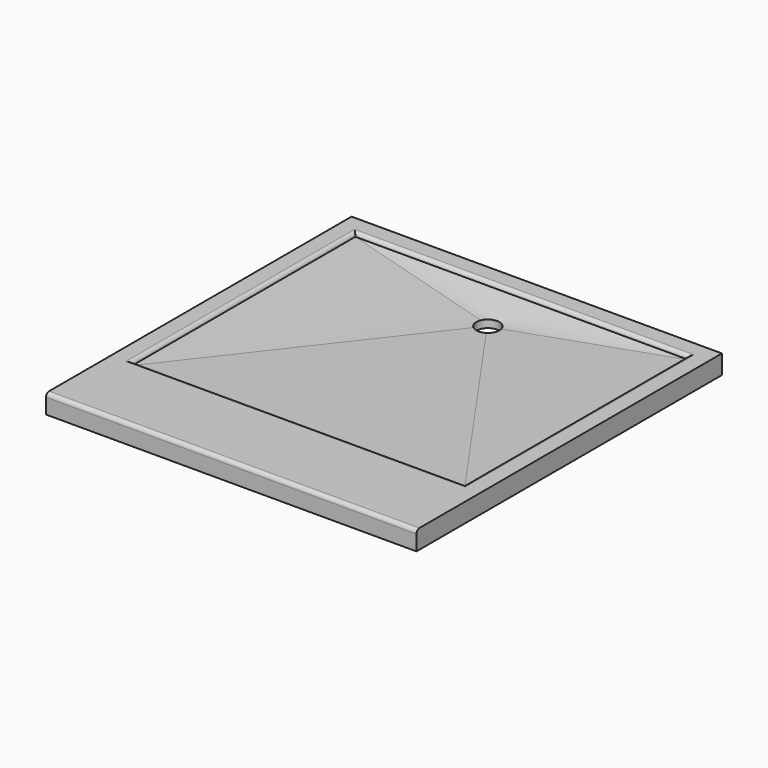
from build123d import *

# Parameters (mm, degrees)
F0_W      = 970
F0_H      = 1000
F1_DEPTH  = 50
F2_W      = 870
F2_H      = 730
F5_DEPTH  = 10
F4_R      = 30
F14_DEPTH = 25
F15_R     = 9.99999


# Not quite as in the source:
# - a fillet or chamfer is up to 0.001 mm smaller than in the source, because OpenCascade refuses the exact size
# - the arcs of a loft's sections are written as splines that run evenly, so that the points pair up as in the source's solid


with BuildPart() as f1:
    # F0 (on Top) → F1 (new body)
    with BuildSketch(Plane.XY):
        Rectangle(F0_W, F0_H)
    extrude(amount=F1_DEPTH)

    # F2 (on face) → F5 (cut)
    with BuildSketch(Plane.XY.offset(50)):
        with Locations((0, 85)):
            Rectangle(F2_W, F2_H)
    extrude(amount=-F5_DEPTH, mode=Mode.SUBTRACT)

    # F12 (on 3pt) → F13 section 0
    with BuildSketch(Plane.XY.offset(40)):
        Polygon((435, -280), (435, 450), (0, 450), (-435, 450), (-435, -280), align=None)
    # F4 (on offset) → F13 section 1
    with BuildSketch(Plane.XY.offset(20)):
        with BuildLine():
            add(Edge.make_bspline(
                [(29.0845037285, 347.3547020923), (28.3143211264, 350.4004242005), (27.0619459332, 353.3236889303), (23.7146117851, 358.6409976204), (21.6201937161, 361.0341823725), (16.7935510128, 365.0568603137), (14.0621063014, 366.6857034902), (8.2286204599, 369.0199829381), (5.1275219455, 369.7250420202), (1.9928685748, 369.9337347293)],
                knots=[0, 0, 0, 0, 0.25, 0.25, 0.5, 0.5, 0.75, 0.75, 1, 1, 1, 1], degree=3))
            add(Edge.make_bspline(
                [(1.9928685748, 369.9337347293), (-1.1417847959, 370.1424274384), (-4.308979984, 369.8546863306), (-10.4004242005, 368.3143211264), (-13.3236889303, 367.0619459332), (-18.6409976204, 363.7146117851), (-21.0341823725, 361.6201937161), (-25.0568603137, 356.7935510128), (-26.6857034902, 354.0621063014), (-27.8528432142, 351.1453633807)],
                knots=[0, 0, 0, 0, 0.25, 0.25, 0.5, 0.5, 0.75, 0.75, 1, 1, 1, 1], degree=3))
            add(Edge.make_bspline(
                [(-27.8528432142, 351.1453633807), (-29.0199829381, 348.2286204599), (-29.7250420202, 345.1275219455), (-30.1424274384, 338.8582152041), (-29.8546863306, 335.691020016), (-28.3143211264, 329.5995757995), (-27.0619459332, 326.6763110697), (-23.7146117851, 321.3590023796), (-21.6201937161, 318.9658176275), (-19.2068723645, 316.9544786569)],
                knots=[0, 0, 0, 0, 0.25, 0.25, 0.5, 0.5, 0.75, 0.75, 1, 1, 1, 1], degree=3))
            add(Edge.make_bspline(
                [(-19.2068723645, 316.9544786569), (-16.7935510128, 314.9431396863), (-14.0621063014, 313.3142965098), (-8.2286204599, 310.9800170619), (-5.1275219455, 310.2749579798), (1.1417847959, 309.8575725616), (4.308979984, 310.1453136694), (10.4004242005, 311.6856788736), (13.3236889303, 312.9380540668), (15.9823432753, 314.6117211409)],
                knots=[0, 0, 0, 0, 0.25, 0.25, 0.5, 0.5, 0.75, 0.75, 1, 1, 1, 1], degree=3))
            add(Edge.make_bspline(
                [(15.9823432753, 314.6117211409), (18.6409976204, 316.2853882149), (21.0341823725, 318.3798062839), (25.0568603137, 323.2064489872), (26.6857034902, 325.9378936986), (29.0199829381, 331.7713795401), (29.7250420202, 334.8724780545), (30.1424274384, 341.1417847959), (29.8546863306, 344.308979984), (29.0845037285, 347.3547020923)],
                knots=[0, 0, 0, 0, 0.25, 0.25, 0.5, 0.5, 0.75, 0.75, 1, 1, 1, 1], degree=3))
        make_face()
    loft(ruled=True, mode=Mode.SUBTRACT)

    # F4 (on offset) → F14 (cut)
    with BuildSketch(Plane.XY.offset(20)):
        with Locations((0, 340)):
            Circle(F4_R)
    extrude(amount=-F14_DEPTH, mode=Mode.SUBTRACT)

    # F15 (radius 10 in the source; OpenCascade refuses exactly that, so slightly less here)
    f15_edges = [f1.edges().sort_by_distance(p)[0] for p in [
        (-435, 85, 50),
        (0, 450, 50),
        (435, 85, 50),
        (0, -280, 50),
        (0, -500, 50),
    ]]
    fillet(f15_edges, radius=F15_R)


solid = f1.part
